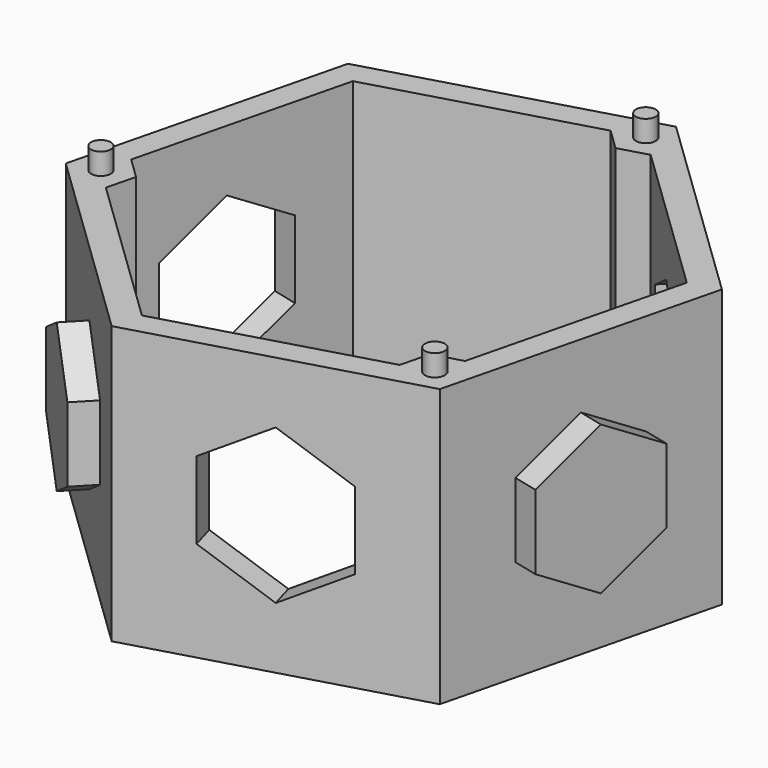
from build123d import *

# Parameters (mm, degrees)
F1_DEPTH  = 32.332
F2_R      = 1.3
F3_DEPTH  = 3.5
F4_R      = 1.15
F5_DEPTH  = 2.5
F12_DEPTH = 3
F13_DEPTH = 3
F14_DEPTH = 3
F15_DEPTH = 3
F16_DEPTH = 3
F17_DEPTH = 3


# Not quite as in the source:
# - a feature names something its author has since deleted; it is built from what else it names


with BuildPart() as f1:
    # F0 (on Top) → F1 (new body)
    with BuildSketch(Plane.XY):
        Polygon((-7.7747095404, -31.3829129447), (23.2910450847, -22.4245524414), (31.0657546251, 8.9583605033), (7.7747095404, 31.3829129447), (-23.2910450847, 22.4245524414), (-31.0657546251, -8.9583605033), align=None)
        Polygon((21.6285805621, -16.6594668643), (20.7955759684, -20.0219218227), (17.4671022586, -20.9817461623), (-6.9417049468, -28.0204579863), (-25.241811799, -10.4011667824), (-27.7372809153, -7.9985361637), (-26.9042763216, -4.6360812053), (-20.7955759684, 20.0219218227), (3.613231237, 27.0606336467), (6.9417049468, 28.0204579863), (9.437174063, 25.6178273676), (27.7372809153, 7.9985361637), align=None, mode=Mode.SUBTRACT)
        Polygon((-27.7372809153, -7.9985361637), (-25.241811799, -10.4011667824), (-24.4088072054, -7.038711824), (-26.9042763216, -4.6360812053), align=None)
        Polygon((6.1087003532, 24.658003028), (9.437174063, 25.6178273676), (6.9417049468, 28.0204579863), (3.613231237, 27.0606336467), align=None)
        Polygon((17.4671022586, -20.9817461623), (20.7955759684, -20.0219218227), (21.6285805621, -16.6594668643), (18.3001068522, -17.619291204), align=None)
    extrude(amount=F1_DEPTH)

    # F2 (on face) → F3 (cut)
    with BuildSketch(Plane(origin=(0, 0, 0), x_dir=(1, 0, 0), z_dir=(0, 0, -1))):
        with Locations((20.7955759684, 20.0219218227)):
            Circle(F2_R)
        with Locations((6.9417049468, -28.0204579863)):
            Circle(F2_R)
        with Locations((-27.7372809153, 7.9985361637)):
            Circle(F2_R)
    extrude(amount=-F3_DEPTH, mode=Mode.SUBTRACT)

    # F4 (on face) → F5 (join)
    with BuildSketch(Plane.XY.offset(32.332)):
        with Locations((6.9417049468, 28.0204579863)):
            Circle(F4_R)
        with Locations((20.7955759684, -20.0219218227)):
            Circle(F4_R)
        with Locations((-27.7372809153, -7.9985361637)):
            Circle(F4_R)
    extrude(amount=F5_DEPTH)

    # F9 (on face) → F12 (join)
    with BuildSketch(Plane(origin=(27.1783998549, -6.7330959691, 0), x_dir=(0.2404677132, 0.9706571377, 0), z_dir=(0.9706571377, -0.2404677132, 0))):
        Polygon((-7.5, 20.4961270189), (-7.5, 11.8358729811), (0, 7.5057459622), (7.5, 11.8358729811), (7.5, 20.4961270189), (0, 24.8262540378), align=None)
    extrude(amount=F12_DEPTH)

    # F7 (on face) → F13 (join)
    with BuildSketch(Plane(origin=(-7.7581677721, 26.9037326931, 0), x_dir=(-0.9608475962, -0.2770774204, 0), z_dir=(-0.2770774204, 0.9608475962, 0))):
        Polygon((-7.5, 20.4961270189), (-7.5, 11.8358729811), (0, 7.5057459622), (7.5, 11.8358729811), (7.5, 20.4961270189), (0, 24.8262540378), align=None)
    extrude(amount=F13_DEPTH)

    # F11 (on face) → F14 (join)
    with BuildSketch(Plane(origin=(-19.4202320828, -20.170636724, 0), x_dir=(0.720379883, -0.6935797172, 0), z_dir=(-0.6935797172, -0.720379883, 0))):
        Polygon((-7.0119504524, 20.4961270189), (-7.0119504524, 11.8358729811), (0.4880495476, 7.5057459622), (7.9880495476, 11.8358729811), (7.9880495476, 20.4961270189), (0.4880495476, 24.8262540378), align=None)
    extrude(amount=F14_DEPTH)

    # F10 (on face) → F15 (cut, through all)
    with BuildSketch(Plane(origin=(7.7581677721, -26.9037326931, 0), x_dir=(0.9608475962, 0.2770774204, 0), z_dir=(0.2770774204, -0.9608475962, 0))):
        Polygon((-7.8, 20.6693320997), (-7.8, 11.6626679003), (0, 7.1593358006), (7.8, 11.6626679003), (7.8, 20.6693320997), (0, 25.1726641994), align=None)
    extrude(amount=-F15_DEPTH, mode=Mode.SUBTRACT)

    # F6 (on face) → F16 (cut, through all)
    with BuildSketch(Plane(origin=(-27.1783998549, 6.7330959691, 0), x_dir=(-0.2404677132, -0.9706571377, 0), z_dir=(-0.9706571377, 0.2404677132, 0))):
        Polygon((-7.8, 20.6693320997), (-7.8, 11.6626679003), (0, 7.1593358006), (7.8, 11.6626679003), (7.8, 20.6693320997), (0, 25.1726641994), align=None)
    extrude(amount=-F16_DEPTH, mode=Mode.SUBTRACT)

    # F8 (on face) → F17 (cut, through all)
    with BuildSketch(Plane(origin=(19.4202320828, 20.170636724, 0), x_dir=(-0.720379883, 0.6935797172, 0), z_dir=(0.6935797172, 0.720379883, 0))):
        Polygon((-7.8, 20.6693320997), (-7.8, 11.6626679003), (0, 7.1593358006), (7.8, 11.6626679003), (7.8, 20.6693320997), (0, 25.1726641994), align=None)
    extrude(amount=-F17_DEPTH, mode=Mode.SUBTRACT)


solid = f1.part
